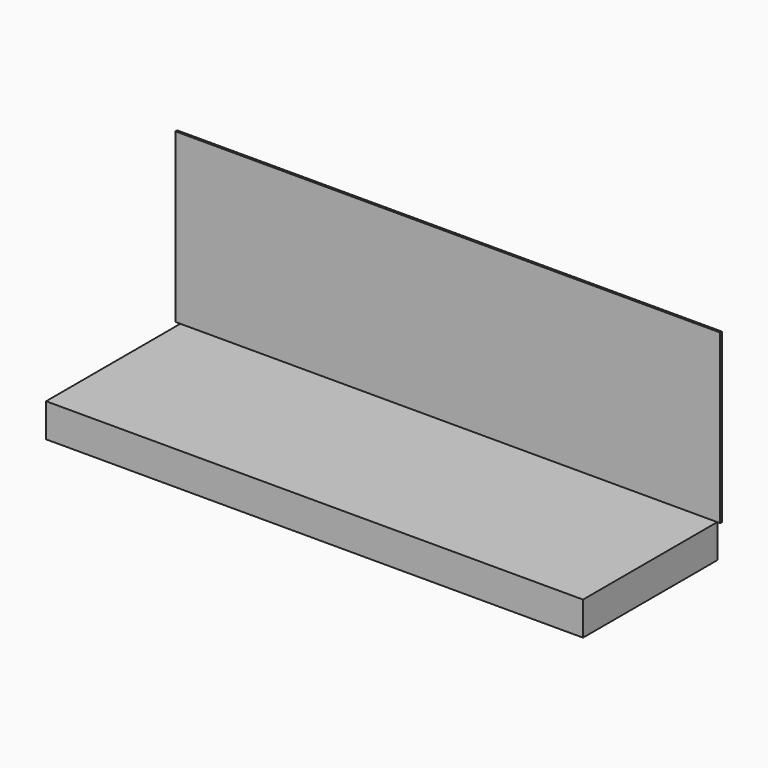
from build123d import *

# Parameters (mm, degrees)
F0_W     = 82.4718438089
F0_H     = 25.4
F1_DEPTH = 0.3302
F4_W     = 81.28
F4_H     = 25.4
F5_DEPTH = 5.08


# Not quite as in the source:
# - the program builds the solid bodies; features that only make, move or delete a surface that nothing else refers to are left out


with BuildPart() as f1:
    # F0 (on Front) → F1 (new body)
    with BuildSketch(Plane.XZ):
        with Locations((3.077307716, 12.7)):
            Rectangle(F0_W, F0_H)
    extrude(amount=-F1_DEPTH)


with BuildPart() as f5:
    # F4 (on Top) → F5 (new body)
    with BuildSketch(Plane.XY):
        with Locations((3.2327694142, -12.7)):
            Rectangle(F4_W, F4_H)
    extrude(amount=-F5_DEPTH)


solid = Compound([f1.part, f5.part])
